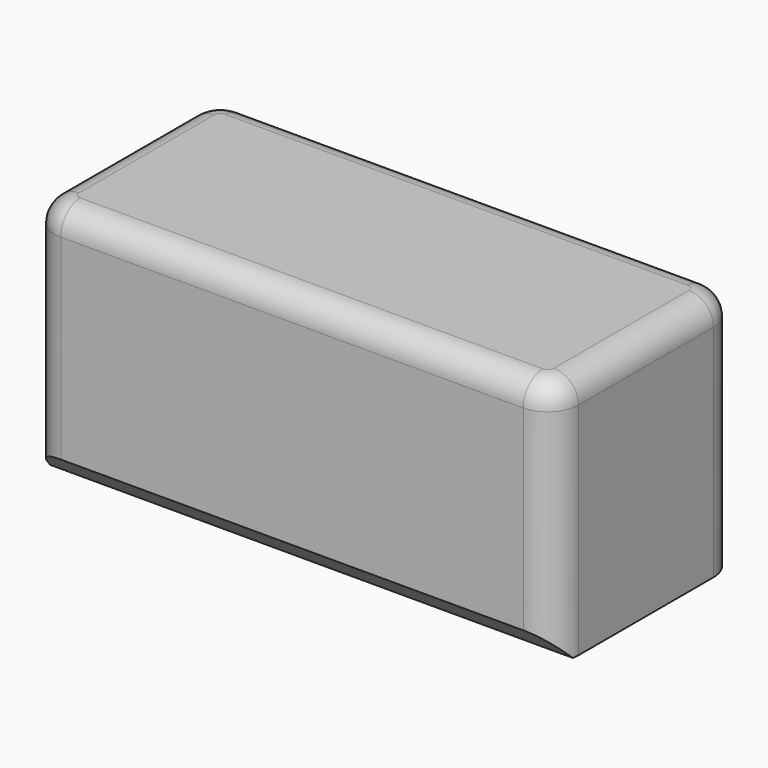
from build123d import *

# Parameters (mm, degrees)
F1_DEPTH      = 25.4
F1_DEPTH_BACK = 25.4
F2_R          = 5.08
F3_T1_DEPTH   = 122.1211277236


# Not quite as in the source:
# - a fillet or chamfer that OpenCascade refuses, or shapes differently, is made with other operations: its cross-section is extruded or revolved along the edge and cut away or added


with BuildPart() as f1:
    # F0 (on Top) → F1 (new body, two sides)
    with BuildSketch(Plane.XY) as f1_sk:
        with BuildLine():
            Line((47.9964142829, 0), (-47.9964142829, 0))
            ThreePointArc((-47.9964142829, 0), (-52.4865423435, -1.8598719395), (-54.3464142829, -6.35))
            Line((-54.3464142829, -6.35), (-54.3464142829, -41.3772979915))
            ThreePointArc((-54.3464142829, -41.3772979915), (-52.4865423435, -45.867426052), (-47.9964142829, -47.7272979915))
            Line((-47.9964142829, -47.7272979915), (47.9964142829, -47.7272979915))
            ThreePointArc((47.9964142829, -47.7272979915), (52.4865423435, -45.867426052), (54.3464142829, -41.3772979915))
            Line((54.3464142829, -41.3772979915), (54.3464142829, -6.35))
            ThreePointArc((54.3464142829, -6.35), (52.4865423435, -1.8598719395), (47.9964142829, 0))
        make_face()
    extrude(amount=F1_DEPTH)
    extrude(f1_sk.sketch, amount=-F1_DEPTH_BACK)

    # F2
    f2_edges = [f1.edges().sort_by_distance(p)[0] for p in [
        (0, -47.727298, 25.4),
        (54.346414, -23.863649, 25.4),
        (-52.486542, -45.867426, 25.4),
        (-54.346414, -23.863649, 25.4),
        (-52.486542, -1.859872, 25.4),
        (0, 0, 25.4),
        (52.486542, -1.859872, 25.4),
        (52.486542, -45.867426, 25.4),
    ]]
    fillet(f2_edges, radius=F2_R)

    # F3: chamfer of 5.08 on 1 edges, made by hand

    # F3_s2 → F3_t1 (cut)
    with BuildSketch(Plane.YZ.offset(-61.0605638618)):
        Polygon((-42.6472979915, -25.4), (-47.7272979915, -20.32), (-47.7272979915, -25.4), align=None)
    extrude(amount=F3_T1_DEPTH, mode=Mode.SUBTRACT)


solid = f1.part
